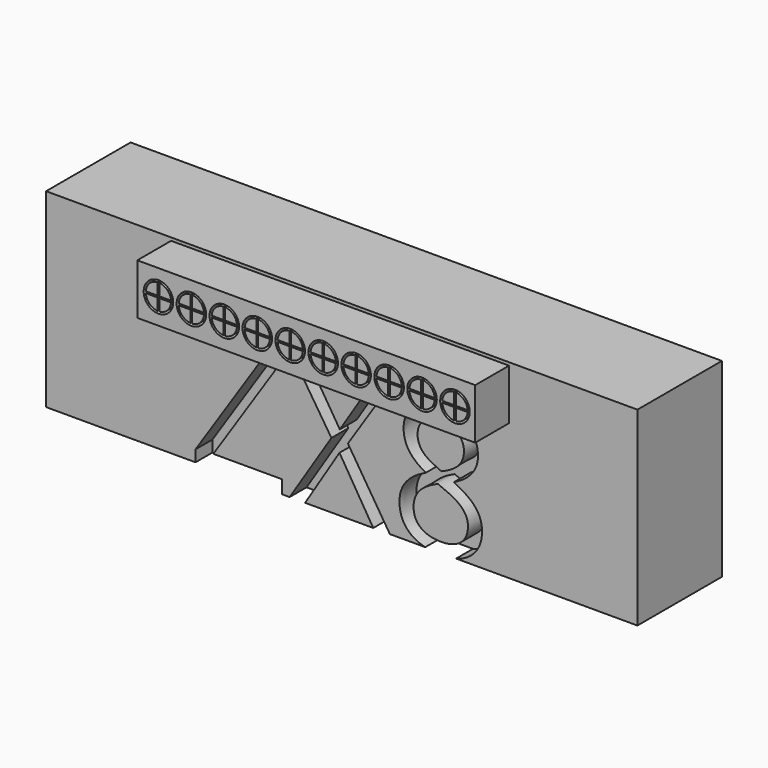
from build123d import *

# Parameters (mm, degrees)
F0_W         = 140
F0_H         = 45
F1_DEPTH     = 25
F2_TEXT_SIZE = 41.6666666667
F3_DEPTH     = 5
F4_W         = 80
F4_H         = 12
F4_R         = 3.5
F5_DEPTH     = 10


# Not quite as in the source:
# - Text() gives the source's letters only with a copy of the font that has no kerning and outlines rounded to 1/6400 em; it was checked with that copy


with BuildPart() as f1:
    # F0 (on Front) → F1 (new body)
    with BuildSketch(Plane.XZ):
        Rectangle(F0_W, F0_H)
    extrude(amount=F1_DEPTH)

    # F2 (on face) → F3 (cut)
    with BuildSketch(Plane.XZ.offset(25)):
        with Locations((-36.2849904693, -22.5)):
            Text('ZX8', F2_TEXT_SIZE, font='Open Sans', text_align=(TextAlign.LEFT, TextAlign.BOTTOM))
    extrude(amount=-F3_DEPTH, mode=Mode.SUBTRACT)

    # F4 (on face) → F5 (join)
    with BuildSketch(Plane.XZ.offset(25)):
        with Locations((-0.3998616919, 15.7884055093)):
            Rectangle(F4_W, F4_H)
        with Locations((-35.3998616919, 15.7884055093)):
            Circle(F4_R, mode=Mode.SUBTRACT)
        with Locations((-27.5998616919, 15.7884055093)):
            Circle(F4_R, mode=Mode.SUBTRACT)
        with Locations((-19.7998616919, 15.7884055093)):
            Circle(F4_R, mode=Mode.SUBTRACT)
        with Locations((-11.9998616919, 15.7884055093)):
            Circle(F4_R, mode=Mode.SUBTRACT)
        with Locations((-4.1998616919, 15.7884055093)):
            Circle(F4_R, mode=Mode.SUBTRACT)
        with Locations((3.6001383081, 15.7884055093)):
            Circle(F4_R, mode=Mode.SUBTRACT)
        with Locations((11.4001383081, 15.7884055093)):
            Circle(F4_R, mode=Mode.SUBTRACT)
        with Locations((19.2001383081, 15.7884055093)):
            Circle(F4_R, mode=Mode.SUBTRACT)
        with Locations((27.0001383081, 15.7884055093)):
            Circle(F4_R, mode=Mode.SUBTRACT)
        with Locations((34.8001383081, 15.7884055093)):
            Circle(F4_R, mode=Mode.SUBTRACT)
        with BuildLine():
            Line((-35.5998616919, 15.9884055093), (-35.5998616919, 18.7817314187))
            ThreePointArc((-35.5998616919, 18.7817314187), (-37.5211820355, 17.9097258529), (-38.3931876014, 15.9884055093))
            Line((-38.3931876014, 15.9884055093), (-35.5998616919, 15.9884055093))
        make_face()
        with BuildLine():
            Line((-35.1998616919, 15.9884055093), (-32.4065357825, 15.9884055093))
            ThreePointArc((-32.4065357825, 15.9884055093), (-33.2785413484, 17.9097258529), (-35.1998616919, 18.7817314187))
            Line((-35.1998616919, 18.7817314187), (-35.1998616919, 15.9884055093))
        make_face()
        with BuildLine():
            ThreePointArc((-35.1998616919, 12.7950795999), (-33.2785413484, 13.6670851657), (-32.4065357825, 15.5884055093))
            Line((-32.4065357825, 15.5884055093), (-35.1998616919, 15.5884055093))
            Line((-35.1998616919, 15.5884055093), (-35.1998616919, 12.7950795999))
        make_face()
        with BuildLine():
            ThreePointArc((-38.3931876014, 15.5884055093), (-37.5211820355, 13.6670851657), (-35.5998616919, 12.7950795999))
            Line((-35.5998616919, 12.7950795999), (-35.5998616919, 15.5884055093))
            Line((-35.5998616919, 15.5884055093), (-38.3931876014, 15.5884055093))
        make_face()
        with BuildLine():
            Line((-27.7998616919, 15.9884055093), (-27.7998616919, 18.7817314187))
            ThreePointArc((-27.7998616919, 18.7817314187), (-29.7211820355, 17.9097258529), (-30.5931876014, 15.9884055093))
            Line((-30.5931876014, 15.9884055093), (-27.7998616919, 15.9884055093))
        make_face()
        with BuildLine():
            Line((-27.3998616919, 15.9884055093), (-24.6065357825, 15.9884055093))
            ThreePointArc((-24.6065357825, 15.9884055093), (-25.4785413484, 17.9097258529), (-27.3998616919, 18.7817314187))
            Line((-27.3998616919, 18.7817314187), (-27.3998616919, 15.9884055093))
        make_face()
        with BuildLine():
            ThreePointArc((-27.3998616919, 12.7950795999), (-25.4785413484, 13.6670851657), (-24.6065357825, 15.5884055093))
            Line((-24.6065357825, 15.5884055093), (-27.3998616919, 15.5884055093))
            Line((-27.3998616919, 15.5884055093), (-27.3998616919, 12.7950795999))
        make_face()
        with BuildLine():
            ThreePointArc((-30.5931876014, 15.5884055093), (-29.7211820355, 13.6670851657), (-27.7998616919, 12.7950795999))
            Line((-27.7998616919, 12.7950795999), (-27.7998616919, 15.5884055093))
            Line((-27.7998616919, 15.5884055093), (-30.5931876014, 15.5884055093))
        make_face()
        with BuildLine():
            ThreePointArc((-22.7931876014, 15.5884055093), (-21.9211820355, 13.6670851657), (-19.9998616919, 12.7950795999))
            Line((-19.9998616919, 12.7950795999), (-19.9998616919, 15.5884055093))
            Line((-19.9998616919, 15.5884055093), (-22.7931876014, 15.5884055093))
        make_face()
        with BuildLine():
            Line((-19.9998616919, 15.9884055093), (-19.9998616919, 18.7817314187))
            ThreePointArc((-19.9998616919, 18.7817314187), (-21.9211820355, 17.9097258529), (-22.7931876014, 15.9884055093))
            Line((-22.7931876014, 15.9884055093), (-19.9998616919, 15.9884055093))
        make_face()
        with BuildLine():
            Line((-19.5998616919, 15.9884055093), (-16.8065357825, 15.9884055093))
            ThreePointArc((-16.8065357825, 15.9884055093), (-17.6785413484, 17.9097258529), (-19.5998616919, 18.7817314187))
            Line((-19.5998616919, 18.7817314187), (-19.5998616919, 15.9884055093))
        make_face()
        with BuildLine():
            ThreePointArc((-19.5998616919, 12.7950795999), (-17.6785413484, 13.6670851657), (-16.8065357825, 15.5884055093))
            Line((-16.8065357825, 15.5884055093), (-19.5998616919, 15.5884055093))
            Line((-19.5998616919, 15.5884055093), (-19.5998616919, 12.7950795999))
        make_face()
        with BuildLine():
            ThreePointArc((-14.9931876014, 15.5884055093), (-14.1211820355, 13.6670851657), (-12.1998616919, 12.7950795999))
            Line((-12.1998616919, 12.7950795999), (-12.1998616919, 15.5884055093))
            Line((-12.1998616919, 15.5884055093), (-14.9931876014, 15.5884055093))
        make_face()
        with BuildLine():
            Line((-12.1998616919, 15.9884055093), (-12.1998616919, 18.7817314187))
            ThreePointArc((-12.1998616919, 18.7817314187), (-14.1211820355, 17.9097258529), (-14.9931876014, 15.9884055093))
            Line((-14.9931876014, 15.9884055093), (-12.1998616919, 15.9884055093))
        make_face()
        with BuildLine():
            Line((-11.7998616919, 15.9884055093), (-9.0065357825, 15.9884055093))
            ThreePointArc((-9.0065357825, 15.9884055093), (-9.8785413484, 17.9097258529), (-11.7998616919, 18.7817314187))
            Line((-11.7998616919, 18.7817314187), (-11.7998616919, 15.9884055093))
        make_face()
        with BuildLine():
            ThreePointArc((-11.7998616919, 12.7950795999), (-9.8785413484, 13.6670851657), (-9.0065357825, 15.5884055093))
            Line((-9.0065357825, 15.5884055093), (-11.7998616919, 15.5884055093))
            Line((-11.7998616919, 15.5884055093), (-11.7998616919, 12.7950795999))
        make_face()
        with BuildLine():
            ThreePointArc((-7.1931876014, 15.5884055093), (-6.3211820355, 13.6670851657), (-4.3998616919, 12.7950795999))
            Line((-4.3998616919, 12.7950795999), (-4.3998616919, 15.5884055093))
            Line((-4.3998616919, 15.5884055093), (-7.1931876014, 15.5884055093))
        make_face()
        with BuildLine():
            Line((-4.3998616919, 15.9884055093), (-4.3998616919, 18.7817314187))
            ThreePointArc((-4.3998616919, 18.7817314187), (-6.3211820355, 17.9097258529), (-7.1931876014, 15.9884055093))
            Line((-7.1931876014, 15.9884055093), (-4.3998616919, 15.9884055093))
        make_face()
        with BuildLine():
            Line((-3.9998616919, 15.9884055093), (-1.2065357825, 15.9884055093))
            ThreePointArc((-1.2065357825, 15.9884055093), (-2.0785413484, 17.9097258529), (-3.9998616919, 18.7817314187))
            Line((-3.9998616919, 18.7817314187), (-3.9998616919, 15.9884055093))
        make_face()
        with BuildLine():
            ThreePointArc((-3.9998616919, 12.7950795999), (-2.0785413484, 13.6670851657), (-1.2065357825, 15.5884055093))
            Line((-1.2065357825, 15.5884055093), (-3.9998616919, 15.5884055093))
            Line((-3.9998616919, 15.5884055093), (-3.9998616919, 12.7950795999))
        make_face()
        with BuildLine():
            ThreePointArc((0.6068123986, 15.5884055093), (1.4788179645, 13.6670851657), (3.4001383081, 12.7950795999))
            Line((3.4001383081, 12.7950795999), (3.4001383081, 15.5884055093))
            Line((3.4001383081, 15.5884055093), (0.6068123986, 15.5884055093))
        make_face()
        with BuildLine():
            Line((3.4001383081, 15.9884055093), (3.4001383081, 18.7817314187))
            ThreePointArc((3.4001383081, 18.7817314187), (1.4788179645, 17.9097258529), (0.6068123986, 15.9884055093))
            Line((0.6068123986, 15.9884055093), (3.4001383081, 15.9884055093))
        make_face()
        with BuildLine():
            Line((3.8001383081, 15.9884055093), (6.5934642175, 15.9884055093))
            ThreePointArc((6.5934642175, 15.9884055093), (5.7214586516, 17.9097258529), (3.8001383081, 18.7817314187))
            Line((3.8001383081, 18.7817314187), (3.8001383081, 15.9884055093))
        make_face()
        with BuildLine():
            ThreePointArc((3.8001383081, 12.7950795999), (5.7214586516, 13.6670851657), (6.5934642175, 15.5884055093))
            Line((6.5934642175, 15.5884055093), (3.8001383081, 15.5884055093))
            Line((3.8001383081, 15.5884055093), (3.8001383081, 12.7950795999))
        make_face()
        with BuildLine():
            Line((11.2001383081, 15.9884055093), (11.2001383081, 18.7817314187))
            ThreePointArc((11.2001383081, 18.7817314187), (9.2788179645, 17.9097258529), (8.4068123986, 15.9884055093))
            Line((8.4068123986, 15.9884055093), (11.2001383081, 15.9884055093))
        make_face()
        with BuildLine():
            Line((11.6001383081, 15.9884055093), (14.3934642175, 15.9884055093))
            ThreePointArc((14.3934642175, 15.9884055093), (13.5214586516, 17.9097258529), (11.6001383081, 18.7817314187))
            Line((11.6001383081, 18.7817314187), (11.6001383081, 15.9884055093))
        make_face()
        with BuildLine():
            ThreePointArc((11.6001383081, 12.7950795999), (13.5214586516, 13.6670851657), (14.3934642175, 15.5884055093))
            Line((14.3934642175, 15.5884055093), (11.6001383081, 15.5884055093))
            Line((11.6001383081, 15.5884055093), (11.6001383081, 12.7950795999))
        make_face()
        with BuildLine():
            ThreePointArc((8.4068123986, 15.5884055093), (9.2788179645, 13.6670851657), (11.2001383081, 12.7950795999))
            Line((11.2001383081, 12.7950795999), (11.2001383081, 15.5884055093))
            Line((11.2001383081, 15.5884055093), (8.4068123986, 15.5884055093))
        make_face()
        with BuildLine():
            Line((19.0001383081, 15.9884055093), (19.0001383081, 18.7817314187))
            ThreePointArc((19.0001383081, 18.7817314187), (17.0788179645, 17.9097258529), (16.2068123986, 15.9884055093))
            Line((16.2068123986, 15.9884055093), (19.0001383081, 15.9884055093))
        make_face()
        with BuildLine():
            Line((19.4001383081, 15.9884055093), (22.1934642175, 15.9884055093))
            ThreePointArc((22.1934642175, 15.9884055093), (21.3214586516, 17.9097258529), (19.4001383081, 18.7817314187))
            Line((19.4001383081, 18.7817314187), (19.4001383081, 15.9884055093))
        make_face()
        with BuildLine():
            ThreePointArc((19.4001383081, 12.7950795999), (21.3214586516, 13.6670851657), (22.1934642175, 15.5884055093))
            Line((22.1934642175, 15.5884055093), (19.4001383081, 15.5884055093))
            Line((19.4001383081, 15.5884055093), (19.4001383081, 12.7950795999))
        make_face()
        with BuildLine():
            ThreePointArc((16.2068123986, 15.5884055093), (17.0788179645, 13.6670851657), (19.0001383081, 12.7950795999))
            Line((19.0001383081, 12.7950795999), (19.0001383081, 15.5884055093))
            Line((19.0001383081, 15.5884055093), (16.2068123986, 15.5884055093))
        make_face()
        with BuildLine():
            Line((26.8001383081, 15.9884055093), (26.8001383081, 18.7817314187))
            ThreePointArc((26.8001383081, 18.7817314187), (24.8788179645, 17.9097258529), (24.0068123986, 15.9884055093))
            Line((24.0068123986, 15.9884055093), (26.8001383081, 15.9884055093))
        make_face()
        with BuildLine():
            Line((27.2001383081, 15.9884055093), (29.9934642175, 15.9884055093))
            ThreePointArc((29.9934642175, 15.9884055093), (29.1214586516, 17.9097258529), (27.2001383081, 18.7817314187))
            Line((27.2001383081, 18.7817314187), (27.2001383081, 15.9884055093))
        make_face()
        with BuildLine():
            ThreePointArc((27.2001383081, 12.7950795999), (29.1214586516, 13.6670851657), (29.9934642175, 15.5884055093))
            Line((29.9934642175, 15.5884055093), (27.2001383081, 15.5884055093))
            Line((27.2001383081, 15.5884055093), (27.2001383081, 12.7950795999))
        make_face()
        with BuildLine():
            ThreePointArc((24.0068123986, 15.5884055093), (24.8788179645, 13.6670851657), (26.8001383081, 12.7950795999))
            Line((26.8001383081, 12.7950795999), (26.8001383081, 15.5884055093))
            Line((26.8001383081, 15.5884055093), (24.0068123986, 15.5884055093))
        make_face()
        with BuildLine():
            Line((34.6001383081, 15.9884055093), (34.6001383081, 18.7817314187))
            ThreePointArc((34.6001383081, 18.7817314187), (32.6788179645, 17.9097258529), (31.8068123986, 15.9884055093))
            Line((31.8068123986, 15.9884055093), (34.6001383081, 15.9884055093))
        make_face()
        with BuildLine():
            Line((35.0001383081, 15.9884055093), (37.7934642175, 15.9884055093))
            ThreePointArc((37.7934642175, 15.9884055093), (36.9214586516, 17.9097258529), (35.0001383081, 18.7817314187))
            Line((35.0001383081, 18.7817314187), (35.0001383081, 15.9884055093))
        make_face()
        with BuildLine():
            ThreePointArc((35.0001383081, 12.7950795999), (36.9214586516, 13.6670851657), (37.7934642175, 15.5884055093))
            Line((37.7934642175, 15.5884055093), (35.0001383081, 15.5884055093))
            Line((35.0001383081, 15.5884055093), (35.0001383081, 12.7950795999))
        make_face()
        with BuildLine():
            ThreePointArc((31.8068123986, 15.5884055093), (32.6788179645, 13.6670851657), (34.6001383081, 12.7950795999))
            Line((34.6001383081, 12.7950795999), (34.6001383081, 15.5884055093))
            Line((34.6001383081, 15.5884055093), (31.8068123986, 15.5884055093))
        make_face()
    extrude(amount=F5_DEPTH)


solid = f1.part
